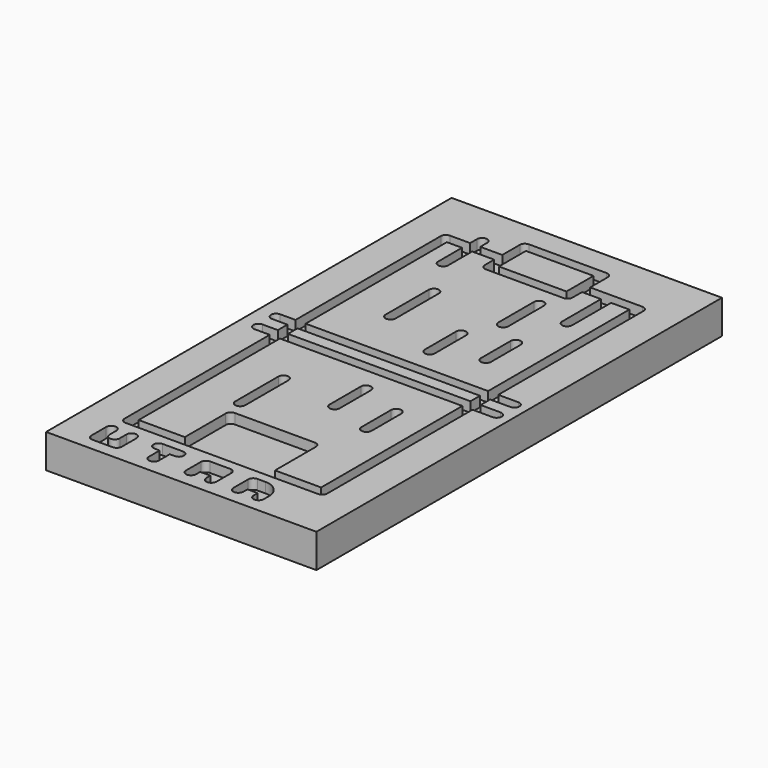
from build123d import *

# Parameters (mm, degrees)
F0_W     = 80
F0_H     = 150
F1_DEPTH = 10
F2_W     = 54
F2_H     = 3.5347917583
F2_W_2   = 20
F2_H_2   = 10
F3_DEPTH = 3
F4_R     = 1.49999
F5_R     = 5.08


# Not quite as in the source:
# - a fillet or chamfer is up to 0.001 mm smaller than in the source, because OpenCascade refuses the exact size


with BuildPart() as f1:
    # F0 (on Top) → F1 (new body)
    with BuildSketch(Plane.XY):
        Rectangle(F0_W, F0_H)
    extrude(amount=F1_DEPTH)

    # F2 (on face) → F3 (cut)
    with BuildSketch(Plane.XY.offset(10)):
        with BuildLine():
            Line((30, 4.7673958791), (30, 60))
            Line((30, 60), (27, 60))
            Line((27, 60), (13, 60))
            Line((13, 60), (13, 65))
            Line((13, 65), (13, 68))
            Line((13, 68), (-13, 68))
            Line((-13, 68), (-13, 60))
            Line((-13, 60), (-19.5125607103, 60))
            Line((-19.5125607103, 60), (-19.5125607103, 62.5778287649))
            ThreePointArc((-19.5125607103, 62.5778287649), (-21.0125607103, 64.0778287649), (-22.5125607103, 62.5778287649))
            Line((-22.5125607103, 62.5778287649), (-22.5125607103, 60))
            Line((-22.5125607103, 60), (-30, 60))
            Line((-30, 60), (-30, 57))
            Line((-30, 57), (-30, 4.7673958791))
            Line((-30, 4.7673958791), (-34.5499739051, 4.7673958791))
            ThreePointArc((-34.5499739051, 4.7673958791), (-36.0499739051, 3.2673958791), (-34.5499739051, 1.7673958791))
            Line((-34.5499739051, 1.7673958791), (-30, 1.7673958791))
            Line((-30, 1.7673958791), (-30, -1.7673958791))
            Line((-30, -1.7673958791), (-34.5499739051, -1.7673958791))
            ThreePointArc((-34.5499739051, -1.7673958791), (-36.0499739051, -3.2673958791), (-34.5499739051, -4.7673958791))
            Line((-34.5499739051, -4.7673958791), (-30, -4.7673958791))
            Line((-30, -4.7673958791), (-30, -60))
            Line((-30, -60), (-27, -60))
            Line((-27, -60), (30, -60))
            Line((30, -60), (30, -57))
            Line((30, -57), (30, -4.7673958791))
            Line((30, -4.7673958791), (35.9570458531, -4.7673958791))
            ThreePointArc((35.9570458531, -4.7673958791), (37.4570458531, -3.2673958791), (35.9570458531, -1.7673958791))
            Line((35.9570458531, -1.7673958791), (30, -1.7673958791))
            Line((30, -1.7673958791), (30, 1.7673958791))
            Line((30, 1.7673958791), (35.9570458531, 1.7673958791))
            ThreePointArc((35.9570458531, 1.7673958791), (37.4570458531, 3.2673958791), (35.9570458531, 4.7673958791))
            Line((35.9570458531, 4.7673958791), (30, 4.7673958791))
        make_face()
        Polygon((-13.3455488831, -57), (-27, -57), (-27, -4.7673958791), (27, -4.7673958791), (27, -57), (13.3455488831, -57), (13.3455488831, -40.3612964153), (-13.3455488831, -40.3612964153), align=None, mode=Mode.SUBTRACT)
        Rectangle(F2_W, F2_H, mode=Mode.SUBTRACT)
        with BuildLine():
            Line((13, 57), (18.5999989513, 57))
            Line((18.5999989513, 57), (18.5999989513, 42.599997338))
            ThreePointArc((18.5999989513, 42.599997338), (20.0999989513, 41.099997338), (21.5999989513, 42.599997338))
            Line((21.5999989513, 42.599997338), (21.5999989513, 57))
            Line((21.5999989513, 57), (27, 57))
            Line((27, 57), (27, 4.7673958791))
            Line((27, 4.7673958791), (-27, 4.7673958791))
            Line((-27, 4.7673958791), (-27, 57))
            Line((-27, 57), (-22.5125607103, 57))
            Line((-22.5125607103, 57), (-22.5125607103, 48.1468625367))
            ThreePointArc((-22.5125607103, 48.1468625367), (-21.0125607103, 46.6468625367), (-19.5125607103, 48.1468625367))
            Line((-19.5125607103, 48.1468625367), (-19.5125607103, 57))
            Line((-19.5125607103, 57), (-13, 57))
            Line((-13, 57), (-13, 52))
            Line((-13, 52), (13, 52))
            Line((13, 52), (13, 57))
        make_face(mode=Mode.SUBTRACT)
        with Locations((0, 60)):
            Rectangle(F2_W_2, F2_H_2, mode=Mode.SUBTRACT)
        with BuildLine():
            ThreePointArc((-27.6987971216, -64.3698275089), (-29.1987971216, -62.8698275089), (-30.6987971216, -64.3698275089))
            Line((-30.6987971216, -64.3698275089), (-30.6987971216, -71.3698275089))
            Line((-30.6987971216, -71.3698275089), (-21.6987971216, -71.3698275089))
            Line((-21.6987971216, -71.3698275089), (-21.6987971216, -64.3698275089))
            ThreePointArc((-21.6987971216, -64.3698275089), (-23.1987971216, -62.8698275089), (-24.6987971216, -64.3698275089))
            Line((-24.6987971216, -64.3698275089), (-24.6987971216, -66.8698275089))
            ThreePointArc((-24.6987971216, -66.8698275089), (-26.1987971216, -68.3698275089), (-27.6987971216, -66.8698275089))
            Line((-27.6987971216, -66.8698275089), (-27.6987971216, -64.3698275089))
        make_face()
        Polygon((-7.6987971216, -62.8698275089), (-16.6987971216, -62.8698275089), (-16.6987971216, -65.8698275089), (-13.6987971216, -65.8698275089), (-13.6987971216, -71.3698275089), (-10.6987971216, -71.3698275089), (-10.6987971216, -65.8698275089), (-7.6987971216, -65.8698275089), align=None)
        Polygon((6.3012028784, -62.8698275089), (-2.6987971216, -62.8698275089), (-2.6987971216, -71.3698275089), (0.3012028784, -71.3698275089), (0.3012028784, -68.3698275089), (3.3012028784, -68.3698275089), (3.3012028784, -71.3698275089), (6.3012028784, -71.3698275089), align=None)
        Polygon((20.3012028784, -62.8698275089), (11.3012028784, -62.8698275089), (11.3012028784, -71.3698275089), (14.3012028784, -71.3698275089), (14.3012028784, -68.3698275089), (17.3012028784, -68.3698275089), (17.3012028784, -71.3698275089), (20.3012028784, -71.3698275089), align=None)
        with BuildLine():
            ThreePointArc((-12.3999991665, 35.8054286294), (-13.8999991665, 37.3054286294), (-15.3999991665, 35.8054286294))
            Line((-15.3999991665, 35.8054286294), (-15.3999991665, 19.805429705))
            ThreePointArc((-15.3999991665, 19.805429705), (-13.8999991665, 18.305429705), (-12.3999991665, 19.805429705))
            Line((-12.3999991665, 19.805429705), (-12.3999991665, 35.8054286294))
        make_face()
        with BuildLine():
            ThreePointArc((10.4000005109, 46.1999991127), (8.9000005109, 47.6999991127), (7.4000005109, 46.1999991127))
            Line((7.4000005109, 46.1999991127), (7.4000005109, 32.9999979834))
            ThreePointArc((7.4000005109, 32.9999979834), (8.9000005109, 31.4999979834), (10.4000005109, 32.9999979834))
            Line((10.4000005109, 32.9999979834), (10.4000005109, 46.1999991127))
        make_face()
        with BuildLine():
            ThreePointArc((5.5999992202, 23.3999986287), (4.0999992202, 24.8999986287), (2.5999992202, 23.3999986287))
            Line((2.5999992202, 23.3999986287), (2.5999992202, 11.7999990051))
            ThreePointArc((2.5999992202, 11.7999990051), (4.0999992202, 10.2999990051), (5.5999992202, 11.7999990051))
            Line((5.5999992202, 11.7999990051), (5.5999992202, 23.3999986287))
        make_face()
        with BuildLine():
            ThreePointArc((18.3999991665, 27.599998548), (16.8999991665, 29.099998548), (15.3999991665, 27.599998548))
            Line((15.3999991665, 27.599998548), (15.3999991665, 16.5999986825))
            ThreePointArc((15.3999991665, 16.5999986825), (16.8999991665, 15.0999986825), (18.3999991665, 16.5999986825))
            Line((18.3999991665, 16.5999986825), (18.3999991665, 27.599998548))
        make_face()
        with BuildLine():
            Line((-12.3999991665, -35.8054286294), (-12.3999991665, -19.805429705))
            ThreePointArc((-12.3999991665, -19.805429705), (-13.8999991665, -18.305429705), (-15.3999991665, -19.805429705))
            Line((-15.3999991665, -19.805429705), (-15.3999991665, -35.8054286294))
            ThreePointArc((-15.3999991665, -35.8054286294), (-13.8999991665, -37.3054286294), (-12.3999991665, -35.8054286294))
        make_face()
        with BuildLine():
            ThreePointArc((5.5999992202, -11.7999990051), (4.0999992202, -10.2999990051), (2.5999992202, -11.7999990051))
            Line((2.5999992202, -11.7999990051), (2.5999992202, -23.3999986287))
            ThreePointArc((2.5999992202, -23.3999986287), (4.0999992202, -24.8999986287), (5.5999992202, -23.3999986287))
            Line((5.5999992202, -23.3999986287), (5.5999992202, -11.7999990051))
        make_face()
        with BuildLine():
            ThreePointArc((18.3999991665, -16.5999986825), (16.8999991665, -15.0999986825), (15.3999991665, -16.5999986825))
            Line((15.3999991665, -16.5999986825), (15.3999991665, -27.599998548))
            ThreePointArc((15.3999991665, -27.599998548), (16.8999991665, -29.099998548), (18.3999991665, -27.599998548))
            Line((18.3999991665, -27.599998548), (18.3999991665, -16.5999986825))
        make_face()
    extrude(amount=-F3_DEPTH, mode=Mode.SUBTRACT)

    # F4 (radius 1.5 in the source; OpenCascade refuses exactly that, so slightly less here)
    f4_edges = [f1.edges().sort_by_distance(p)[0] for p in [
        (-13, 52, 8.5),
        (-13, 68, 8.5),
        (13, 68, 8.5),
        (13, 52, 8.5),
        (30, -60, 8.5),
        (-30, -60, 8.5),
        (-13.345549, -40.361296, 8.5),
        (13.345549, -40.361296, 8.5),
        (-30.698797, -71.369828, 8.5),
        (-21.698797, -71.369828, 8.5),
        (-10.698797, -71.369828, 8.5),
        (-7.698797, -65.869828, 8.5),
        (-13.698797, -71.369828, 8.5),
        (-16.698797, -65.869828, 8.5),
        (-16.698797, -62.869828, 8.5),
        (-7.698797, -62.869828, 8.5),
        (6.301203, -62.869828, 8.5),
        (-2.698797, -62.869828, 8.5),
        (11.301203, -62.869828, 8.5),
        (20.301203, -71.369828, 8.5),
        (14.301203, -71.369828, 8.5),
        (6.301203, -71.369828, 8.5),
        (0.301203, -71.369828, 8.5),
        (17.301203, -71.369828, 8.5),
        (11.301203, -71.369828, 8.5),
        (-2.698797, -71.369828, 8.5),
        (3.301203, -71.369828, 8.5),
        (-30, 60, 8.5),
        (30, 60, 8.5),
    ]]
    fillet(f4_edges, radius=F4_R)

    # F5
    f5_edges = [f1.edges().sort_by_distance(p)[0] for p in [
        (20.301203, -62.869828, 8.5),
    ]]
    fillet(f5_edges, radius=F5_R)


solid = f1.part
